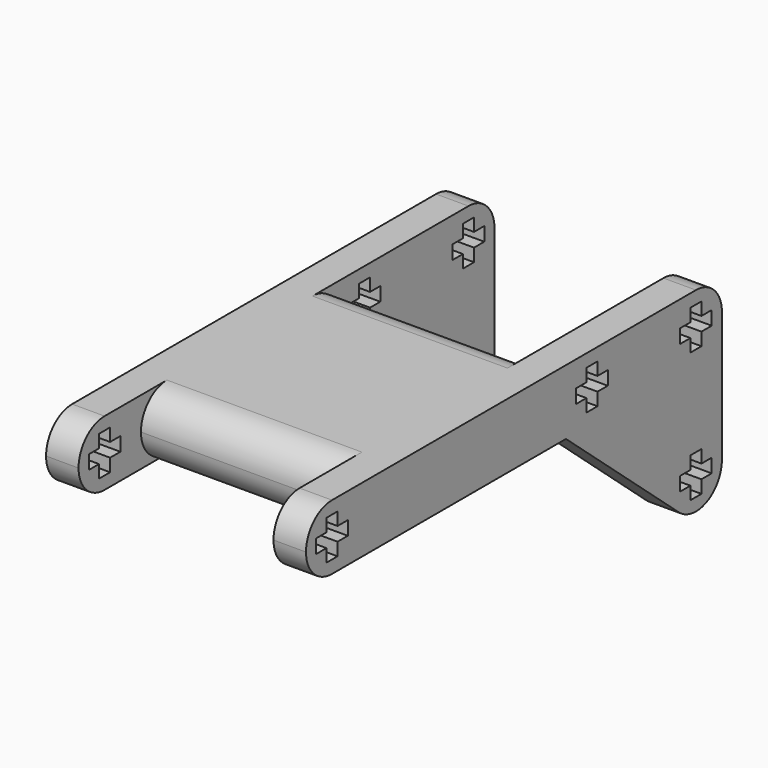
from build123d import *

# Parameters (mm, degrees)
F1_DEPTH = 7.9375
F2_R     = 3.96874
F3_W     = 3.96875
F3_H     = 23.8125
F4_DEPTH = 15.875
F5_W     = 1.56845
F5_H     = 1.6891
F5_W_2   = 1.6891
F5_H_2   = 1.56845
F6_DEPTH = 31.75


# Not quite as in the source:
# - a fillet or chamfer is up to 0.001 mm smaller than in the source, because OpenCascade refuses the exact size


with BuildPart() as f1:
    # F0 (on Top) → F1 (new body)
    with BuildSketch(Plane.XY):
        Polygon((0, 63.5), (0, 0), (3.96875, 0), (3.96875, 9.525), (27.78125, 9.525), (27.78125, 0), (31.75, 0), (31.75, 63.5), (27.78125, 63.5), (27.78125, 39.6875), (3.96875, 39.6875), (3.96875, 63.5), align=None)
    extrude(amount=F1_DEPTH)

    # F2 (radius 3.96875 in the source; OpenCascade refuses exactly that, so slightly less here)
    f2_edges = [f1.edges().sort_by_distance(p)[0] for p in [
        (15.875, 39.6875, 7.9375),
        (15.875, 39.6875, 0),
        (1.984375, 63.5, 7.9375),
        (29.765625, 63.5, 7.9375),
        (1.984375, 0, 7.9375),
        (1.984375, 0, 0),
        (29.765625, 0, 7.9375),
        (29.765625, 0, 0),
        (15.875, 9.525, 7.9375),
        (15.875, 9.525, 0),
    ]]
    fillet(f2_edges, radius=F2_R)

    # F3 (on face) → F4 (join)
    with BuildSketch(Plane(origin=(0, 0, 0), x_dir=(1, 0, 0), z_dir=(0, 0, -1))):
        with Locations((29.765625, -51.59375)):
            Rectangle(F3_W, F3_H)
        with Locations((1.984375, -51.59375)):
            Rectangle(F3_W, F3_H)
    extrude(amount=F4_DEPTH)

    # F5 (on face) → F6 (cut, through all)
    with BuildSketch(Plane(origin=(0, 0, 0), x_dir=(0, -1, 0), z_dir=(-1, 0, 0))):
        with Locations((-5.597525, 3.96875)):
            Rectangle(F5_W, F5_H)
        with Locations((-3.96875, 3.96875)):
            Rectangle(F5_W_2, F5_H)
        with Locations((-3.96875, 2.339975)):
            Rectangle(F5_W_2, F5_H_2)
        with Locations((-2.339975, 3.96875)):
            Rectangle(F5_W, F5_H)
        with Locations((-3.96875, 5.597525)):
            Rectangle(F5_W_2, F5_H_2)
        with BuildLine():
            Line((-63.5, -15.875), (-59.53125, -15.875))
            ThreePointArc((-59.53125, -15.875), (-62.3375800378, -14.7125800378), (-63.5, -11.90625))
            Line((-63.5, -11.90625), (-63.5, -15.875))
        make_face()
        with BuildLine():
            Line((-59.53125, -15.875), (-39.6875, -15.875))
            Line((-39.6875, -15.875), (-39.6875, 0))
            Line((-39.6875, 0), (-56.935957382, -14.9088210299))
            ThreePointArc((-56.935957382, -14.9088210299), (-58.146597916, -15.6256202651), (-59.53125, -15.875))
        make_face()
        with Locations((-57.902475, -11.90625)):
            Rectangle(F5_W, F5_H)
        with Locations((-59.53125, -11.90625)):
            Rectangle(F5_W_2, F5_H)
        with Locations((-59.53125, -10.277475)):
            Rectangle(F5_W_2, F5_H_2)
        with Locations((-61.160025, -11.90625)):
            Rectangle(F5_W, F5_H)
        with Locations((-59.53125, -13.535025)):
            Rectangle(F5_W_2, F5_H_2)
        with Locations((-59.53125, 5.597525)):
            Rectangle(F5_W_2, F5_H_2)
        with Locations((-59.53125, 3.96875)):
            Rectangle(F5_W_2, F5_H)
        with Locations((-61.160025, 3.96875)):
            Rectangle(F5_W, F5_H)
        with Locations((-57.902475, 3.96875)):
            Rectangle(F5_W, F5_H)
        with Locations((-59.53125, 2.339975)):
            Rectangle(F5_W_2, F5_H_2)
        with Locations((-43.65625, 5.597525)):
            Rectangle(F5_W_2, F5_H_2)
        with Locations((-43.65625, 3.96875)):
            Rectangle(F5_W_2, F5_H)
        with Locations((-45.285025, 3.96875)):
            Rectangle(F5_W, F5_H)
        with Locations((-42.027475, 3.96875)):
            Rectangle(F5_W, F5_H)
        with Locations((-43.65625, 2.339975)):
            Rectangle(F5_W_2, F5_H_2)
    extrude(amount=-F6_DEPTH, mode=Mode.SUBTRACT)


solid = f1.part
